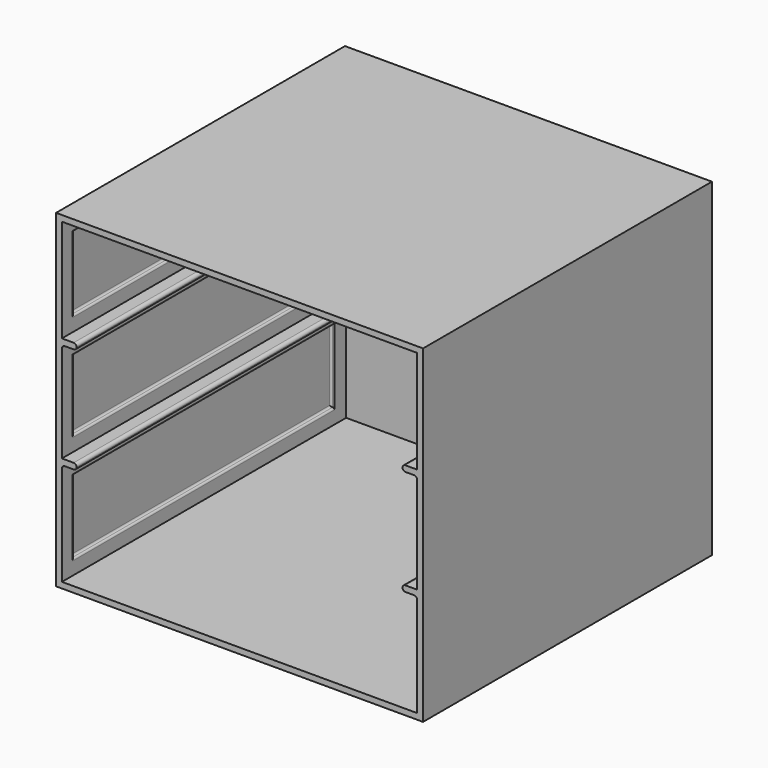
from build123d import *

# Parameters (mm, degrees)
F0_W      = 125
F0_H      = 122
F1_DEPTH  = 2
F2_W      = 121
F2_H      = 2
F2_W_2    = 2
F2_H_2    = 120
F3_DEPTH  = 108
F4_W      = 125
F4_H      = 122
F5_DEPTH  = 2
F6_W      = 4.9999992847
F6_H      = 1
F6_W_2    = 5
F7_DEPTH  = 120
F8_DEPTH  = 1
F9_W      = 111
F9_H      = 25
F9_W_2    = 111.000007391
F9_H_2    = 24.000007391
F9_W_3    = 111.0000030398
F9_H_3    = 25.0000030398
F11_DEPTH = 1.2
F10_W     = 111
F10_H     = 25
F10_H_2   = 24
F12_DEPTH = 1.2
F13_R     = 0.99999
F14_R     = 0.59999


# Not quite as in the source:
# - a fillet or chamfer is up to 0.001 mm smaller than in the source, because OpenCascade refuses the exact size
# - a feature names something its author has since deleted; it is built from what else it names


with BuildPart() as f1:
    # F0 (on Top) → F1 (new body)
    with BuildSketch(Plane.XY):
        Rectangle(F0_W, F0_H)
    extrude(amount=F1_DEPTH)

    # F2 (on face) → F3 (join)
    with BuildSketch(Plane.XY.offset(2)):
        with Locations((0, 60)):
            Rectangle(F2_W, F2_H)
        with Locations((-61.5, 60)):
            Rectangle(F2_W_2, F2_H)
        with Locations((-61.5, -1)):
            Rectangle(F2_W_2, F2_H_2)
        with Locations((61.5, -1)):
            Rectangle(F2_W_2, F2_H_2)
        with Locations((61.5, 60)):
            Rectangle(F2_W_2, F2_H)
    extrude(amount=F3_DEPTH)

    # F4 (on face) → F5 (join)
    with BuildSketch(Plane.XY.offset(110)):
        Rectangle(F4_W, F4_H)
    extrude(amount=F5_DEPTH)

    # F6 (on face) → F7 (join)
    with BuildSketch(Plane.XZ.offset(61)):
        with Locations((-58.0000003576, 74.5)):
            Rectangle(F6_W, F6_H)
        with Locations((-58.0000003576, 73.5)):
            Rectangle(F6_W, F6_H)
        with Locations((-58.0000003576, 38.5)):
            Rectangle(F6_W, F6_H)
        with Locations((-58.0000003576, 37.5)):
            Rectangle(F6_W, F6_H)
        with Locations((58, 74.5)):
            Rectangle(F6_W_2, F6_H)
        with Locations((58, 73.5)):
            Rectangle(F6_W_2, F6_H)
        with Locations((58, 38.5)):
            Rectangle(F6_W_2, F6_H)
        with Locations((58, 37.5)):
            Rectangle(F6_W_2, F6_H)
    extrude(amount=-F7_DEPTH)

    # F8 (add): a face of the model
    f8_faces = [f1.faces().sort_by_distance(p)[0] for p in [
        (-60.821637703, -61, 56),
    ]]
    extrude(f8_faces, amount=F8_DEPTH)

    # F9 (on face) → F11 (cut)
    with BuildSketch(Plane.YZ.offset(-60.5)):
        with Locations((-1.5, 92.5)):
            Rectangle(F9_W, F9_H)
        with Locations((-1.5, 56)):
            Rectangle(F9_W_2, F9_H_2)
        with Locations((-1.5, 19.5)):
            Rectangle(F9_W_3, F9_H_3)
    extrude(amount=-F11_DEPTH, mode=Mode.SUBTRACT)

    # F10 (on face) → F12 (cut)
    with BuildSketch(Plane(origin=(60.5, 0, 0), x_dir=(0, -1, 0), z_dir=(-1, 0, 0))):
        with Locations((1.5, 92.5)):
            Rectangle(F10_W, F10_H)
        with Locations((1.5, 56)):
            Rectangle(F10_W, F10_H_2)
        with Locations((1.5, 19.5)):
            Rectangle(F10_W, F10_H)
    extrude(amount=-F12_DEPTH, mode=Mode.SUBTRACT)

    # F13 (radius 1 in the source; OpenCascade refuses exactly that, so slightly less here)
    f13_edges = [f1.edges().sort_by_distance(p)[0] for p in [
        (55.5, -1.5, 75),
        (55.5, -1.5, 73),
        (55.5, -1.5, 39),
        (55.5, -1.5, 37),
        (-55.500001, -1.5, 75),
        (-55.500001, -1.5, 73),
        (-55.500001, -1.5, 39),
        (-55.500001, -1.5, 37),
        (-60.5, -1.5, 73),
        (-60.5, -1.5, 37),
        (60.5, -1.5, 73),
        (60.5, -1.5, 37),
    ]]
    fillet(f13_edges, radius=F13_R)

    # F14 (radius 0.6 in the source; OpenCascade refuses exactly that, so slightly less here)
    f14_edges = [f1.edges().sort_by_distance(p)[0] for p in [
        (-61.7, 54, 92.5),
        (-61.7, -1.5, 105),
        (-61.7, -57, 92.5),
        (-61.7, -1.5, 80),
        (-60.5, -1.5, 80),
        (-60.5, -57, 92.5),
        (-60.5, -1.5, 105),
        (-60.5, 54, 92.5),
        (-61.7, 54.000004, 56),
        (-61.7, -1.5, 68.000004),
        (-61.7, -57.000004, 56),
        (-61.7, -1.5, 43.999996),
        (-60.5, -1.5, 68.000004),
        (-60.5, -57.000004, 56),
        (-60.5, 54.000004, 56),
        (-60.5, -1.5, 43.999996),
        (-61.7, -1.5, 6.999998),
        (-61.7, 54.000002, 19.5),
        (-61.7, -1.5, 32.000002),
        (-61.7, -57.000002, 19.5),
        (-60.5, -1.5, 32.000002),
        (-60.5, -57.000002, 19.5),
        (-60.5, -1.5, 6.999998),
        (61.7, -57, 19.5),
        (61.7, -1.5, 32),
        (61.7, 54, 19.5),
        (61.7, -1.5, 7),
        (61.7, -1.5, 68),
        (61.7, 54, 56),
        (61.7, -1.5, 44),
        (61.7, -57, 56),
        (61.7, -1.5, 105),
        (61.7, 54, 92.5),
        (61.7, -1.5, 80),
        (61.7, -57, 92.5),
        (60.5, -1.5, 105),
        (60.5, 54, 92.5),
        (60.5, -57, 92.5),
        (61.1, 54, 80),
        (61.1, -57, 80),
        (60.5, -1.5, 80),
        (60.5, -1.5, 68),
        (60.5, -57, 56),
        (60.5, 54, 56),
        (60.5, -1.5, 44),
        (60.5, 54, 19.5),
        (60.5, -1.5, 32),
        (60.5, -1.5, 7),
        (60.5, -57, 19.5),
    ]]
    fillet(f14_edges, radius=F14_R)


solid = f1.part
